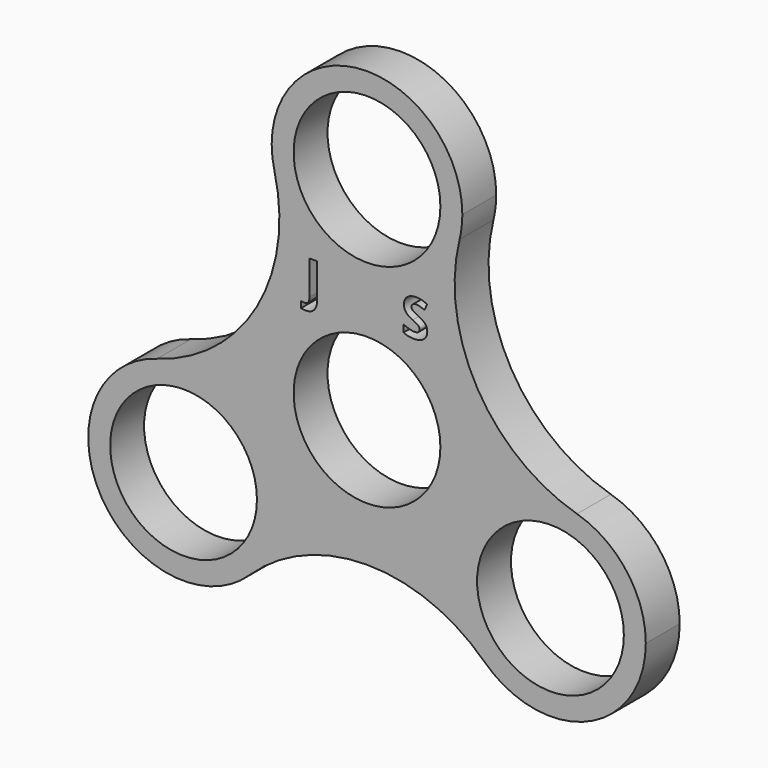
from build123d import *

# Parameters (mm, degrees)
F1_R         = 14.2875
F1_R_2       = 10.9982
F2_DEPTH     = 6.35
F3_TEXT_SIZE = 7.6421722673
F4_DEPTH     = 25.4
F0_R         = 14.2875
F0_R_2       = 10.9982
F5_DEPTH     = 6.35


# Not quite as in the source:
# - Text() gives the source's letters only with a copy of the font that has no kerning and outlines rounded to 1/6400 em; it was checked with that copy


with BuildPart() as f2:
    # F1 (on Front) → F2 (new body)
    with BuildSketch(Plane.XZ):
        with BuildLine():
            ThreePointArc((31.4695122777, -2.1510686152), (16.5359438351, 9.5470316245), (13.8718760728, 28.3289313848))
            ThreePointArc((13.8718760728, 28.3289313848), (0, 17.4625), (-13.8718760728, 28.3289313848))
            ThreePointArc((-13.8718760728, 28.3289313848), (-16.5359438351, 9.5470316245), (-31.4695122777, -2.1510686152))
            ThreePointArc((-31.4695122777, -2.1510686152), (-18.912441482, -4.4535326513), (-13.2088065702, -15.875))
            ThreePointArc((-13.2088065702, -15.875), (-14.3517276668, -21.4743483284), (-17.5976362049, -26.1778627696))
            ThreePointArc((-17.5976362049, -26.1778627696), (0, -19.094063249), (17.5976362049, -26.1778627696))
            ThreePointArc((17.5976362049, -26.1778627696), (15.1229686136, -8.73125), (31.4695122777, -2.1510686152))
        make_face()
        Circle(F1_R, mode=Mode.SUBTRACT)
        with BuildLine():
            ThreePointArc((-13.8718760728, 28.3289313848), (0, 17.4625), (13.8718760728, 28.3289313848))
            ThreePointArc((13.8718760728, 28.3289313848), (14.1832134166, 30.0268884454), (14.2875, 31.75))
            ThreePointArc((14.2875, 31.75), (-1.7231115546, 45.9332134166), (-13.8718760728, 28.3289313848))
        make_face()
        with Locations((0, 31.75)):
            Circle(F1_R_2, mode=Mode.SUBTRACT)
        with BuildLine():
            ThreePointArc((41.7838065702, -15.875), (38.9177739189, -7.2911349119), (31.4695122777, -2.1510686152))
            ThreePointArc((31.4695122777, -2.1510686152), (15.1229686136, -8.73125), (17.5976362049, -26.1778627696))
            ThreePointArc((17.5976362049, -26.1778627696), (33.0956548986, -29.0195789034), (41.7838065702, -15.875))
        make_face()
        with Locations((27.4963065702, -15.875)):
            Circle(F1_R_2, mode=Mode.SUBTRACT)
        with BuildLine():
            ThreePointArc((-13.2088065702, -15.875), (-18.912441482, -4.4535326513), (-31.4695122777, -2.1510686152))
            ThreePointArc((-31.4695122777, -2.1510686152), (-39.8696445267, -23.01875), (-17.5976362049, -26.1778627696))
            ThreePointArc((-17.5976362049, -26.1778627696), (-14.3517276668, -21.4743483284), (-13.2088065702, -15.875))
        make_face()
        with Locations((-27.4963065702, -15.875)):
            Circle(F1_R_2, mode=Mode.SUBTRACT)
    extrude(amount=F2_DEPTH)

    # F3 (on face) → F4 (cut)
    with BuildSketch(Plane.XZ.offset(6.35)):
        with Locations((-9.3229890912, 13.0681134411)):
            Text('J      S', F3_TEXT_SIZE, font='Open Sans', font_style=FontStyle.BOLD, text_align=(TextAlign.LEFT, TextAlign.BOTTOM))
    extrude(amount=-F4_DEPTH, mode=Mode.SUBTRACT)

    # F0 (on Front) → F5 (join)
    with BuildSketch(Plane.XZ):
        Circle(F0_R)
        Circle(F0_R_2, mode=Mode.SUBTRACT)
    extrude(amount=F5_DEPTH)


solid = f2.part
